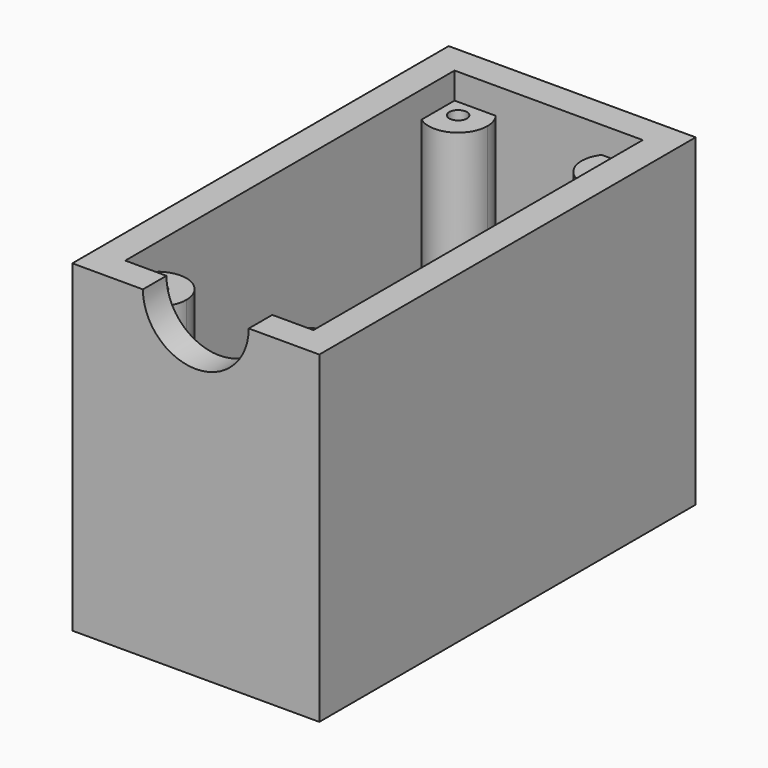
from build123d import *

# Parameters (mm, degrees)
F0_W     = 21
F0_H     = 40
F1_DEPTH = 25
F0_R     = 0.75
F2_DEPTH = 22.75
F3_W     = 21
F3_H     = 40
F4_DEPTH = 2.5
F5_R     = 4.5
F6_DEPTH = 2.5


# Not quite as in the source:
# - a feature names something its author has since deleted; it is built from what else it names


with BuildPart() as f1:
    # F0 (on Top) → F1 (new body)
    with BuildSketch(Plane.XY):
        Rectangle(F0_W, F0_H)
        with BuildLine():
            ThreePointArc((-8, 13.996502206), (-8.2693131131, 17.7627216453), (-4.5026281309, 17.5))
            Line((-4.5026281309, 17.5), (4.5026281309, 17.5))
            ThreePointArc((4.5026281309, 17.5), (7.2926444119, 18.3675177766), (9, 15.996502206))
            ThreePointArc((9, 15.996502206), (8.7360679775, 14.8784682172), (8, 13.996502206))
            Line((8, 13.996502206), (8, -13.9965024172))
            ThreePointArc((8, -13.9965024172), (8.7360679775, -14.8784684285), (9, -15.9965024172))
            ThreePointArc((9, -15.9965024172), (7.2926442865, -18.3675180298), (4.5026279719, -17.5))
            Line((4.5026279719, -17.5), (-4.4973814273, -17.5))
            ThreePointArc((-4.4973814273, -17.5), (-8.2662214687, -17.7728088813), (-8, -14.003497794))
            Line((-8, -14.003497794), (-8, 13.996502206))
        make_face(mode=Mode.SUBTRACT)
        with BuildLine():
            Line((-8, -17.5), (-8, -14.003497794))
            ThreePointArc((-8, -14.003497794), (-8.2662214687, -17.7728088813), (-4.4973814273, -17.5))
            Line((-4.4973814273, -17.5), (-8, -17.5))
        make_face()
        with BuildLine():
            Line((-8, 13.996502206), (-8, 17.5))
            Line((-8, 17.5), (-4.5026281309, 17.5))
            ThreePointArc((-4.5026281309, 17.5), (-8.2693131131, 17.7627216453), (-8, 13.996502206))
        make_face()
        with BuildLine():
            ThreePointArc((9, 15.996502206), (7.2926444119, 18.3675177766), (4.5026281309, 17.5))
            Line((4.5026281309, 17.5), (8, 17.5))
            Line((8, 17.5), (8, 13.996502206))
            ThreePointArc((8, 13.996502206), (8.7360679775, 14.8784682172), (9, 15.996502206))
        make_face()
        with BuildLine():
            ThreePointArc((9, -15.9965024172), (8.7360679775, -14.8784684285), (8, -13.9965024172))
            Line((8, -13.9965024172), (8, -17.5))
            Line((8, -17.5), (4.5026279719, -17.5))
            ThreePointArc((4.5026279719, -17.5), (7.2926442865, -18.3675180298), (9, -15.9965024172))
        make_face()
    extrude(amount=F1_DEPTH)

    # F0 (on Top) → F2 (join)
    with BuildSketch(Plane.XY):
        with BuildLine():
            Line((-4.5026281309, 17.5), (-8, 17.5))
            Line((-8, 17.5), (-8, 13.996502206))
            ThreePointArc((-8, 13.996502206), (-5.3819660113, 13.7604342285), (-4, 15.996502206))
            ThreePointArc((-4, 15.996502206), (-4.1289844293, 16.7891466178), (-4.5026281309, 17.5))
        make_face()
        with Locations((-6.5, 15.996502206)):
            Circle(F0_R, mode=Mode.SUBTRACT)
        with BuildLine():
            Line((8, 17.5), (4.5026281309, 17.5))
            ThreePointArc((4.5026281309, 17.5), (4.7306868869, 14.2302827667), (8, 13.996502206))
            Line((8, 13.996502206), (8, 17.5))
        make_face()
        with Locations((6.5, 15.996502206)):
            Circle(F0_R, mode=Mode.SUBTRACT)
        with BuildLine():
            Line((8, -17.5), (8, -13.9965024172))
            ThreePointArc((8, -13.9965024172), (4.7306869803, -14.2302828844), (4.5026279719, -17.5))
            Line((4.5026279719, -17.5), (8, -17.5))
        make_face()
        with Locations((6.5, -15.9965024172)):
            Circle(F0_R, mode=Mode.SUBTRACT)
        with BuildLine():
            ThreePointArc((-4, -16.003497794), (-5.3819660113, -13.7674298165), (-8, -14.003497794))
            Line((-8, -14.003497794), (-8, -17.5))
            Line((-8, -17.5), (-4.4973814273, -17.5))
            ThreePointArc((-4.4973814273, -17.5), (-4.1276018007, -16.7919943281), (-4, -16.003497794))
        make_face()
        with Locations((-6.5, -16.003497794)):
            Circle(F0_R, mode=Mode.SUBTRACT)
    extrude(amount=F2_DEPTH)

    # F3 (on face) → F4 (join)
    with BuildSketch(Plane.XY):
        Rectangle(F3_W, F3_H)
    extrude(amount=-F4_DEPTH)

    # F5 (on face) → F6 (cut)
    with BuildSketch(Plane.XZ.offset(20)):
        with Locations((0, 25)):
            Circle(F5_R)
    extrude(amount=-F6_DEPTH, mode=Mode.SUBTRACT)


solid = f1.part
